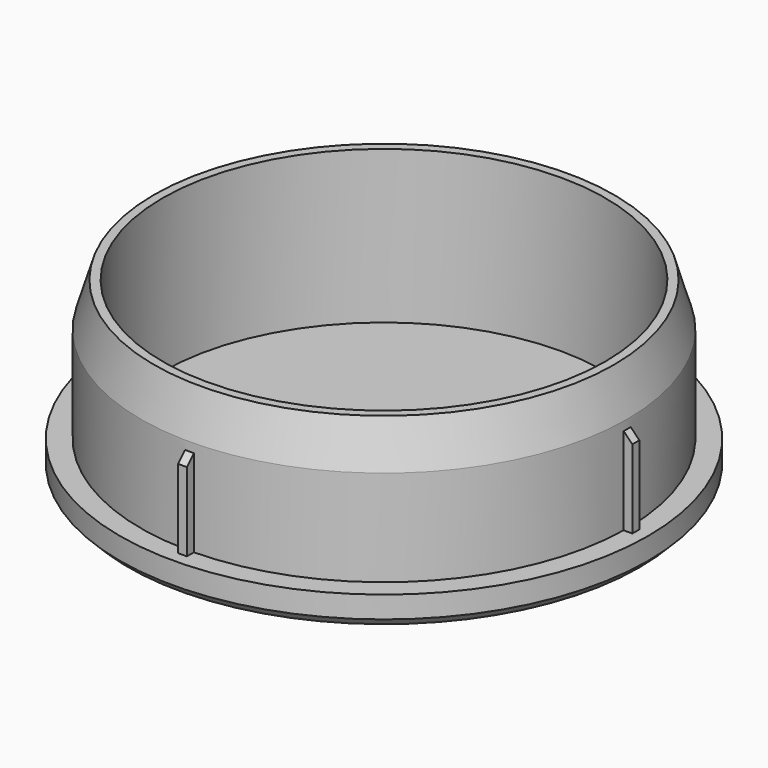
from build123d import *

# Parameters (mm, degrees)
F0_R      = 30.25
F1_DEPTH  = 3.5
F3_R      = 27.85
F3_R_2    = 25.35
F4_DEPTH  = 10
F5_DEPTH  = 6
F6_SIZE2  = 1.5
F6_SIZE   = 5
F8_DEPTH  = 10
F9_SIZE   = 0.99999
F10_DEPTH = 1.5
F11_SIZE  = 1


# Not quite as in the source:
# - a fillet or chamfer is up to 0.001 mm smaller than in the source, because OpenCascade refuses the exact size


with BuildPart() as f1:
    # F0 (on Top) → F1 (new body)
    with BuildSketch(Plane.XY):
        Circle(F0_R)
    extrude(amount=F1_DEPTH)

    # F3 (on face) → F4 (join)
    with BuildSketch(Plane.XY.offset(3.5)):
        Circle(F3_R)
        Circle(F3_R_2, mode=Mode.SUBTRACT)
    extrude(amount=F4_DEPTH)

    # F5 (add): a face of the model
    f5_faces = [f1.faces().sort_by_distance(p)[0] for p in [
        (-27.0622830458, 0, 13.5),
    ]]
    extrude(f5_faces, amount=F5_DEPTH)

    # F6
    f6_edges = [f1.edges().sort_by_distance(p)[0] for p in [
        (-27.85, 0, 19.5),
    ]]
    f6_side = f1.faces().sort_by_distance((-27.85, 0, 11.5))[0]
    chamfer(f6_edges, length=F6_SIZE, length2=F6_SIZE2, reference=f6_side)

    # F7 (on face) → F8 (join)
    with BuildSketch(Plane.XY.offset(3.5)):
        with BuildLine():
            ThreePointArc((27.85, 0), (27.8488778044, -0.250010074), (27.8455113079, -0.5))
            Line((27.8455113079, -0.5), (28.85, -0.5))
            Line((28.85, -0.5), (28.85, 0.5))
            Line((28.85, 0.5), (27.8455113079, 0.5))
            ThreePointArc((27.8455113079, 0.5), (27.8488778044, 0.250010074), (27.85, 0))
        make_face()
        with BuildLine():
            Line((-28.85, -0.5), (-27.8455113079, -0.5))
            ThreePointArc((-27.8455113079, -0.5), (-27.85, 0), (-27.8455113079, 0.5))
            Line((-27.8455113079, 0.5), (-28.85, 0.5))
            Line((-28.85, 0.5), (-28.85, -0.5))
        make_face()
        with BuildLine():
            Line((-0.5, -28.85), (0.5, -28.85))
            Line((0.5, -28.85), (0.5, -27.8455113079))
            ThreePointArc((0.5, -27.8455113079), (0, -27.85), (-0.5, -27.8455113079))
            Line((-0.5, -27.8455113079), (-0.5, -28.85))
        make_face()
        with BuildLine():
            ThreePointArc((-0.5, 27.8455113079), (0, 27.85), (0.5, 27.8455113079))
            Line((0.5, 27.8455113079), (0.5, 28.85))
            Line((0.5, 28.85), (-0.5, 28.85))
            Line((-0.5, 28.85), (-0.5, 27.8455113079))
        make_face()
    extrude(amount=F8_DEPTH)

    # F9 (size 1 in the source; OpenCascade refuses exactly that, so slightly less here)
    f9_edges = [f1.edges().sort_by_distance(p)[0] for p in [
        (28.85, 0, 13.5),
        (0, 28.85, 13.5),
        (-28.85, 0, 13.5),
        (0, -28.85, 13.5),
    ]]
    chamfer(f9_edges, length=F9_SIZE)

    # F10 (cut): a face of the model
    f10_faces = [f1.faces().sort_by_distance(p)[0] for p in [
        (0, 0, 3.5),
    ]]
    extrude(f10_faces, amount=-F10_DEPTH, mode=Mode.SUBTRACT)

    # F11
    f11_edges = [f1.edges().sort_by_distance(p)[0] for p in [
        (-30.25, 0, 0),
    ]]
    chamfer(f11_edges, length=F11_SIZE)


solid = f1.part
